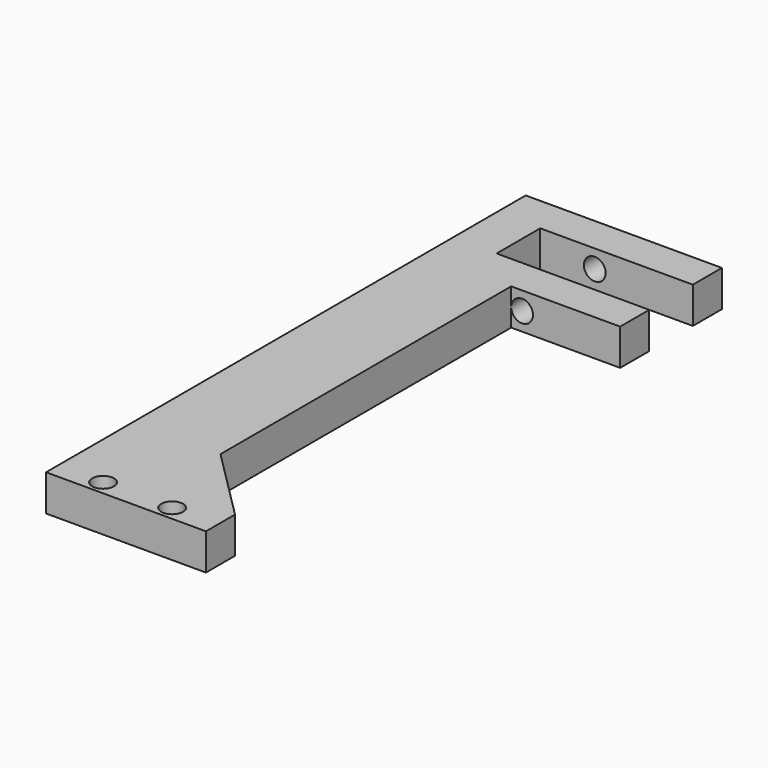
from build123d import *

# Parameters (mm, degrees)
F0_R     = 1.5
F1_DEPTH = 5
F2_SIZE  = 9.99999
F4_DEPTH = 25


# Not quite as in the source:
# - a fillet or chamfer is up to 0.001 mm smaller than in the source, because OpenCascade refuses the exact size


with BuildPart() as f1:
    # F0 (on Top) → F1 (new body)
    with BuildSketch(Plane.XY):
        Polygon((0, 7.5), (0, 0), (0, -75), (11, -75), (22, -75), (22, -60), (12, -60), (12, -10), (27, -10), (27, -5), (6, -5), (6, 2.5), (27, 2.5), (27, 7.5), align=None)
        with Locations((6.25, -73)):
            Circle(F0_R, mode=Mode.SUBTRACT)
        with BuildLine():
            ThreePointArc((17.25, -73), (15.75, -74.5), (14.25, -73))
            ThreePointArc((14.25, -73), (15.75, -71.5), (17.25, -73))
        make_face(mode=Mode.SUBTRACT)
    extrude(amount=F1_DEPTH)

    # F2 (size 10 in the source; OpenCascade refuses exactly that, so slightly less here)
    f2_edges = [f1.edges().sort_by_distance(p)[0] for p in [
        (22, -60, 2.5),
    ]]
    chamfer(f2_edges, length=F2_SIZE)

    # F3 (on face) → F4 (cut)
    with BuildSketch(Plane(origin=(0, 7.5, 0), x_dir=(-1, 0, 0), z_dir=(0, 1, 0))):
        with BuildLine():
            ThreePointArc((-15, 2.5), (-13.5, 1), (-12, 2.5))
            Line((-12, 2.5), (-15, 2.5))
        make_face()
        with BuildLine():
            Line((-15, 2.5), (-12, 2.5))
            ThreePointArc((-12, 2.5), (-13.5, 4), (-15, 2.5))
        make_face()
    extrude(amount=-F4_DEPTH, mode=Mode.SUBTRACT)


solid = f1.part
